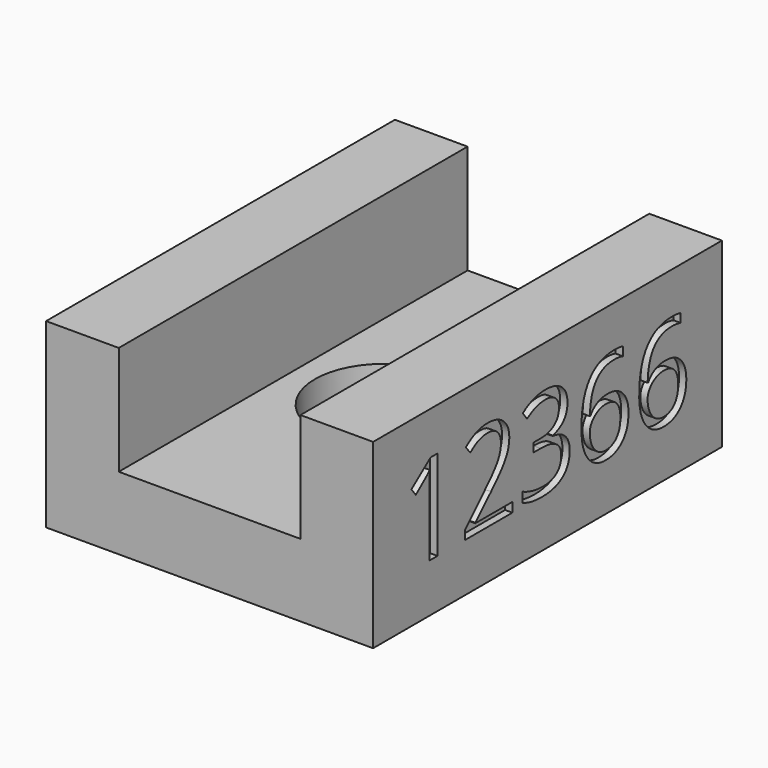
from build123d import *

# Parameters (mm, degrees)
F1_DEPTH     = 60
F2_TEXT_SIZE = 17.3931949125
F3_DEPTH     = 1
F5_DEPTH     = 5.5


# Not quite as in the source:
# - Text() gives the source's letters only with a copy of the font that has no kerning and outlines rounded to 1/6400 em; it was checked with that copy


with BuildPart() as f1:
    # F0 (on Front) → F1 (new body)
    with BuildSketch(Plane.XZ):
        Polygon((-22.5, -12.5), (22.5, -12.5), (22.5, 12.5), (12.5, 12.5), (12.5, -2.5), (-12.5, -2.5), (-12.5, 12.5), (-22.5, 12.5), align=None)
    extrude(amount=F1_DEPTH)

    # F2 (on face) → F3 (cut)
    with BuildSketch(Plane.YZ.offset(22.5)):
        with Locations((-55, -5.8142967637)):
            Text('12366', F2_TEXT_SIZE, font='Open Sans', text_align=(TextAlign.LEFT, TextAlign.BOTTOM))
    extrude(amount=-F3_DEPTH, mode=Mode.SUBTRACT)

    # F4 (on face) → F5 (cut)
    with BuildSketch(Plane.XY.offset(-2.5)):
        with BuildLine():
            Line((0, -39.5), (0, -20.5))
            ThreePointArc((0, -20.5), (-9.5, -30), (0, -39.5))
        make_face()
        with BuildLine():
            ThreePointArc((9.5, -30), (6.7175144213, -23.2824855787), (0, -20.5))
            Line((0, -20.5), (0, -39.5))
            ThreePointArc((0, -39.5), (6.7175144213, -36.7175144213), (9.5, -30))
        make_face()
    extrude(amount=-F5_DEPTH, mode=Mode.SUBTRACT)


solid = f1.part
